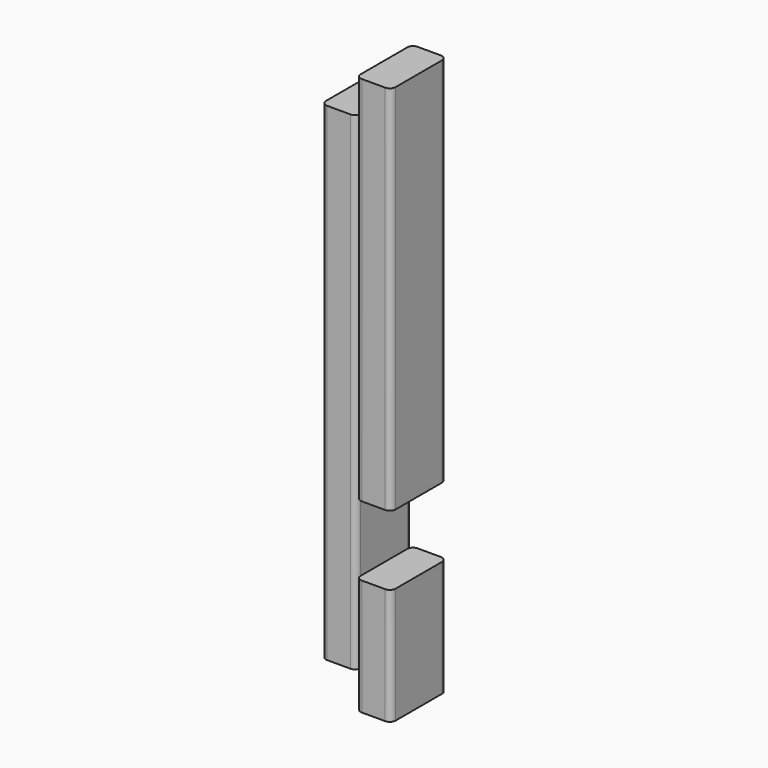
from build123d import *

# Parameters (mm, degrees)
F1_DEPTH = 304.8
F2_DEPTH = 285.75
F3_DEPTH = 19.05
F4_W     = 19.05
F4_H     = 38.1
F5_DEPTH = 38.101


# Not quite as in the source:
# - a feature names something its author has since deleted; it is built from what else it names


with BuildPart() as f1:
    # F0 (on Top) → F1 (new body)
    with BuildSketch(Plane.XY):
        with BuildLine():
            Line((19.05, 34.9504), (19.05, 3.1496))
            ThreePointArc((19.05, 3.1496), (19.972496482, 0.922496482), (22.1996, 0))
            Line((22.1996, 0), (34.9504, 0))
            ThreePointArc((34.9504, 0), (37.177503518, 0.922496482), (38.1, 3.1496))
            Line((38.1, 3.1496), (38.1, 34.9504))
            ThreePointArc((38.1, 34.9504), (37.177503518, 37.177503518), (34.9504, 38.1))
            Line((34.9504, 38.1), (22.1996, 38.1))
            ThreePointArc((22.1996, 38.1), (19.972496482, 37.177503518), (19.05, 34.9504))
        make_face()
    extrude(amount=F1_DEPTH)

    # F0 (on Top) → F2 (join)
    with BuildSketch(Plane.XY):
        with BuildLine():
            ThreePointArc((0, 3.1496), (0.922496482, 0.922496482), (3.1496, 0))
            Line((3.1496, 0), (15.9004, 0))
            ThreePointArc((15.9004, 0), (18.127503518, 0.922496482), (19.05, 3.1496))
            Line((19.05, 3.1496), (19.05, 34.9504))
            ThreePointArc((19.05, 34.9504), (18.127503518, 37.177503518), (15.9004, 38.1))
            Line((15.9004, 38.1), (3.1496, 38.1))
            ThreePointArc((3.1496, 38.1), (0.922496482, 37.177503518), (0, 34.9504))
            Line((0, 34.9504), (0, 3.1496))
        make_face()
        with BuildLine():
            Line((19.05, 34.9504), (19.05, 3.1496))
            ThreePointArc((19.05, 3.1496), (19.972496482, 0.922496482), (22.1996, 0))
            Line((22.1996, 0), (34.9504, 0))
            ThreePointArc((34.9504, 0), (37.177503518, 0.922496482), (38.1, 3.1496))
            Line((38.1, 3.1496), (38.1, 34.9504))
            ThreePointArc((38.1, 34.9504), (37.177503518, 37.177503518), (34.9504, 38.1))
            Line((34.9504, 38.1), (22.1996, 38.1))
            ThreePointArc((22.1996, 38.1), (19.972496482, 37.177503518), (19.05, 34.9504))
        make_face()
    extrude(amount=F2_DEPTH)

    # F0 (on Top) → F3 (cut)
    with BuildSketch(Plane.XY):
        with BuildLine():
            ThreePointArc((0, 3.1496), (0.922496482, 0.922496482), (3.1496, 0))
            Line((3.1496, 0), (15.9004, 0))
            ThreePointArc((15.9004, 0), (18.127503518, 0.922496482), (19.05, 3.1496))
            Line((19.05, 3.1496), (19.05, 34.9504))
            ThreePointArc((19.05, 34.9504), (18.127503518, 37.177503518), (15.9004, 38.1))
            Line((15.9004, 38.1), (3.1496, 38.1))
            ThreePointArc((3.1496, 38.1), (0.922496482, 37.177503518), (0, 34.9504))
            Line((0, 34.9504), (0, 3.1496))
        make_face()
    extrude(amount=F3_DEPTH, mode=Mode.SUBTRACT)

    # F4 (on face) → F5 (cut, through all)
    with BuildSketch(Plane.XZ):
        with Locations((28.575, 82.55)):
            Rectangle(F4_W, F4_H)
    extrude(amount=-F5_DEPTH, mode=Mode.SUBTRACT)


solid = f1.part
